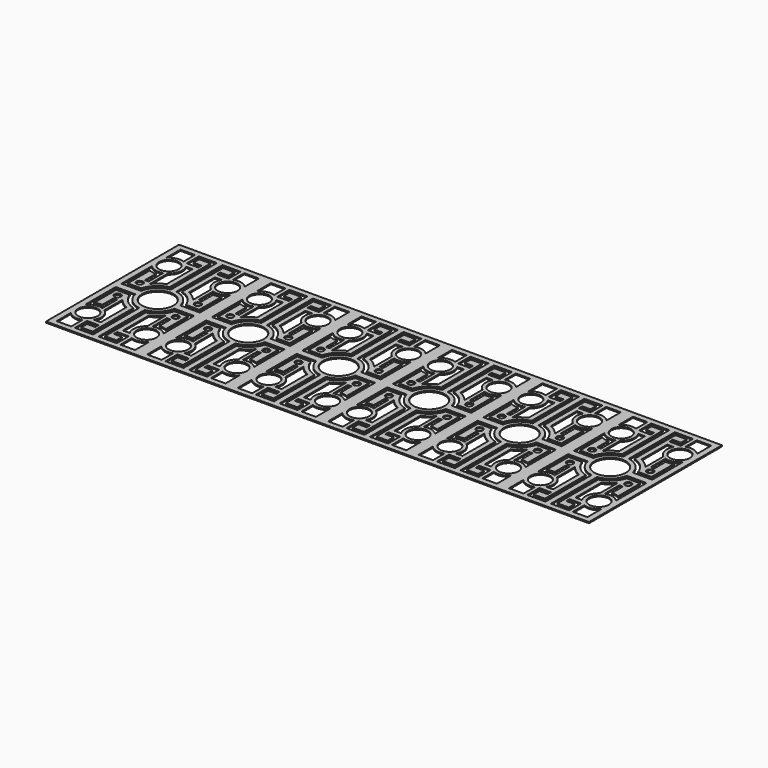
from build123d import *

# Parameters (mm, degrees)
F0_W     = 114.6567612886
F0_H     = 210.6409370899
F0_R     = 12.4910197192
F0_R_2   = 4.1467921194
F1_DEPTH = 1.5


# Not quite as in the source:
# - ends of sketch curves that miss each other by under 0.0002 mm in the source are joined


with BuildPart() as f1:
    # F0 (on Top) → F1 (new body)
    with BuildSketch(Plane.XY):
        with Locations((-114.6567612886, 0)):
            Rectangle(F0_W, F0_H)
        with BuildLine():
            Line((-145.8713209915, -98.179930827), (-164.2948761574, -98.1799308277))
            Line((-164.2948761574, -98.1799308277), (-164.2948761582, -75.6368151295))
            ThreePointArc((-164.2948761582, -75.6368151295), (-155.7558124319, -80.6535810623), (-145.871320992, -80.0372543739))
            Line((-145.871320992, -80.0372543739), (-145.8713209915, -98.179930827))
        make_face(mode=Mode.SUBTRACT)
        with BuildLine():
            Line((-65.0186464199, -98.1799308277), (-83.4422015858, -98.179930827))
            Line((-83.4422015858, -98.179930827), (-83.4422015853, -80.0372543739))
            ThreePointArc((-83.4422015853, -80.0372543739), (-73.5577101454, -80.6535810623), (-65.0187125643, -75.6367543837))
            Line((-65.0187125643, -75.6367543837), (-65.0186464199, -98.1799308277))
        make_face(mode=Mode.SUBTRACT)
        with Locations((-151.8214292036, -64.1815741605)):
            Circle(F0_R, mode=Mode.SUBTRACT)
        with Locations((-77.4920933736, -64.1815741605)):
            Circle(F0_R, mode=Mode.SUBTRACT)
        with BuildLine():
            Line((-118.1285301959, -98.179930827), (-141.0917807374, -98.179930827))
            Line((-141.0917807374, -98.179930827), (-141.0917807374, -79.0647952815))
            Line((-141.0917807374, -79.0647952815), (-126.454948448, -79.0647952815))
            Line((-126.454948448, -79.0647952815), (-126.454948448, -84.2922343872))
            Line((-126.454948448, -84.2922343872), (-136.8864420805, -84.2922343872))
            Line((-136.8864420805, -84.2922343872), (-136.8864420805, -93.5049741529))
            Line((-136.8864420805, -93.5049741529), (-122.577030212, -93.5049741529))
            Line((-122.577030212, -93.5049741529), (-122.4740208728, -28.733128465))
            ThreePointArc((-122.4740208728, -28.733128465), (-135.1857456354, -21.520110379), (-142.9105009887, -9.1127040796))
            Line((-142.9105009887, -9.1127040796), (-160.0093394521, -9.1127040796))
            Line((-160.0093394521, -9.1127040796), (-160.0093394521, -44.1508456133))
            ThreePointArc((-160.0093394521, -44.1508456133), (-155.5141858376, -42.8593906698), (-150.8465334777, -42.5639531376))
            Line((-150.8465334777, -42.5639531376), (-150.8465334777, -25.0186747871))
            Line((-150.8465334777, -25.0186747871), (-146.2718600365, -25.0186747871))
            Line((-146.2718600365, -25.0186747871), (-146.2718600365, -48.3131796792))
            ThreePointArc((-146.2718600365, -48.3131796792), (-155.9772603886, -47.8925370951), (-164.2948761582, -52.9114019158))
            Line((-164.2948761582, -52.9114019158), (-164.2948761582, -4.6059023589))
            Line((-164.2948761582, -4.6059023589), (-139.4034866247, -4.6059023589))
            ThreePointArc((-139.4034866247, -4.6059023589), (-132.0747762414, -18.2690053755), (-118.1285301959, -25.0434131848))
            Line((-118.1285301959, -25.0434131848), (-118.1285301959, -98.179930827))
        make_face(mode=Mode.SUBTRACT)
        with BuildLine():
            Line((-128.7834886465, -72.9014551434), (-137.3203646393, -72.9014551437))
            ThreePointArc((-137.3203646393, -72.9014551437), (-135.2508292753, -60.7563127289), (-141.9659890239, -50.4270295761))
            Line((-141.9659890239, -50.4270295761), (-141.9659890239, -21.7546069546))
            ThreePointArc((-141.9659890239, -21.7546069546), (-135.9951180955, -27.664926491), (-128.7834011022, -31.9747193718))
            Line((-128.7834011022, -31.9747193718), (-128.7834886465, -72.9014551434))
        make_face(mode=Mode.SUBTRACT)
        with BuildLine():
            Line((-92.4270804968, -93.5049741529), (-92.4270804968, -84.2922343872))
            Line((-92.4270804968, -84.2922343872), (-102.8585741293, -84.2922343872))
            Line((-102.8585741293, -84.2922343872), (-102.8585741293, -79.0647952815))
            Line((-102.8585741293, -79.0647952815), (-88.2217418399, -79.0647952815))
            Line((-88.2217418399, -79.0647952815), (-88.2217418399, -98.179930827))
            Line((-88.2217418399, -98.179930827), (-111.1849923813, -98.179930827))
            Line((-111.1849923813, -98.179930827), (-111.1849923813, -25.0434131848))
            ThreePointArc((-111.1849923813, -25.0434131848), (-97.2387463359, -18.2690053755), (-89.9100359526, -4.6059023589))
            Line((-89.9100359526, -4.6059023589), (-65.018646419, -4.6059023589))
            Line((-65.018646419, -4.6059023589), (-65.018646419, -52.9114019158))
            ThreePointArc((-65.018646419, -52.9114019158), (-73.3362621887, -47.8925370951), (-83.0416625408, -48.3131796792))
            Line((-83.0416625408, -48.3131796792), (-83.0416625408, -25.0186747871))
            Line((-83.0416625408, -25.0186747871), (-78.4669890996, -25.0186747871))
            Line((-78.4669890996, -25.0186747871), (-78.4669890996, -42.5639531376))
            ThreePointArc((-78.4669890996, -42.5639531376), (-73.7993367396, -42.8593906698), (-69.3041831251, -44.1508456133))
            Line((-69.3041831251, -44.1508456133), (-69.3041831251, -9.1127040796))
            Line((-69.3041831251, -9.1127040796), (-86.4030215886, -9.1127040796))
            ThreePointArc((-86.4030215886, -9.1127040796), (-94.1277769419, -21.520110379), (-106.8395017045, -28.733128465))
            Line((-106.8395017045, -28.733128465), (-106.7364923652, -93.5049741529))
            Line((-106.7364923652, -93.5049741529), (-92.4270804968, -93.5049741529))
        make_face(mode=Mode.SUBTRACT)
        with BuildLine():
            ThreePointArc((-87.3475335534, -50.4270295761), (-94.062693302, -60.7563127289), (-91.993157938, -72.9014551437))
            Line((-91.993157938, -72.9014551437), (-100.5300339308, -72.9014551434))
            Line((-100.5300339308, -72.9014551434), (-100.5300339308, -31.9747193718))
            ThreePointArc((-100.5300339308, -31.9747193718), (-93.3184044818, -27.664926491), (-87.3475335534, -21.7546069546))
            Line((-87.3475335534, -21.7546069546), (-87.3475335534, -50.4270295761))
        make_face(mode=Mode.SUBTRACT)
        with Locations((-151.4818519357, -17.5733412616)):
            Circle(F0_R_2, mode=Mode.SUBTRACT)
        with Locations((-77.8316706415, -17.5733412616)):
            Circle(F0_R_2, mode=Mode.SUBTRACT)
        with BuildLine():
            ThreePointArc((-134.3588686144, 2.5716374978), (-114.6567612886, 19.8692313011), (-94.9546539628, 2.5716374978))
            ThreePointArc((-94.9546539628, 2.5716374978), (-94.8172855837, 1.2286792521), (-94.7714255579, -0.1205070876))
            ThreePointArc((-94.7714255579, -0.1205070876), (-100.5966835989, -14.1758679), (-114.6567612886, -19.9897318622))
            ThreePointArc((-114.6567612886, -19.9897318622), (-129.6388295453, -13.1897947203), (-134.3588686144, 2.5716374978))
        make_face(mode=Mode.SUBTRACT)
        with Locations((-151.4979563653, 17.452834174)):
            Circle(F0_R_2, mode=Mode.SUBTRACT)
        with Locations((-77.8155662119, 17.452834174)):
            Circle(F0_R_2, mode=Mode.SUBTRACT)
        with BuildLine():
            ThreePointArc((-141.9820934535, 50.3065224885), (-135.2669337049, 60.6358056413), (-137.3364690689, 72.7809480561))
            Line((-137.3364690689, 72.7809480561), (-128.7995930761, 72.7809480559))
            Line((-128.7995930761, 72.7809480559), (-128.7995930761, 31.8542122842))
            ThreePointArc((-128.7995930761, 31.8542122842), (-136.0112225251, 27.5444194035), (-141.9820934535, 21.634099867))
            Line((-141.9820934535, 21.634099867), (-141.9820934535, 50.3065224885))
        make_face(mode=Mode.SUBTRACT)
        with BuildLine():
            Line((-136.9025465101, 93.3844670653), (-136.9025465101, 84.1717272997))
            Line((-136.9025465101, 84.1717272997), (-126.4710528776, 84.1717272997))
            Line((-126.4710528776, 84.1717272997), (-126.4710528776, 78.9442881942))
            Line((-126.4710528776, 78.9442881942), (-141.107885167, 78.9442881942))
            Line((-141.107885167, 78.9442881942), (-141.107885167, 98.0594237397))
            Line((-141.107885167, 98.0594237397), (-118.1446346255, 98.0594237397))
            Line((-118.1446346255, 98.0594237397), (-118.1446346255, 24.9229060972))
            ThreePointArc((-118.1446346255, 24.9229060972), (-132.090880671, 18.1484982879), (-139.4195910543, 4.4853952713))
            Line((-139.4195910543, 4.4853952713), (-164.3109805878, 4.4853952713))
            Line((-164.3109805878, 4.4853952713), (-164.3109805878, 52.7908948282))
            ThreePointArc((-164.3109805878, 52.7908948282), (-155.9933648182, 47.7720300076), (-146.2879644661, 48.1926725917))
            Line((-146.2879644661, 48.1926725917), (-146.2879644661, 24.8981676996))
            Line((-146.2879644661, 24.8981676996), (-150.8626379073, 24.8981676996))
            Line((-150.8626379073, 24.8981676996), (-150.8626379073, 42.44344605))
            ThreePointArc((-150.8626379073, 42.44344605), (-155.5302902672, 42.7388835823), (-160.0254438818, 44.0303385258))
            Line((-160.0254438818, 44.0303385258), (-160.0254438818, 8.992196992))
            Line((-160.0254438818, 8.992196992), (-142.9266054183, 8.992196992))
            ThreePointArc((-142.9266054183, 8.992196992), (-135.201850065, 21.3996032915), (-122.4901253024, 28.6126213774))
            Line((-122.4901253024, 28.6126213774), (-122.5931346416, 93.3844670653))
            Line((-122.5931346416, 93.3844670653), (-136.9025465101, 93.3844670653))
        make_face(mode=Mode.SUBTRACT)
        with BuildLine():
            Line((-100.5139295012, 72.7809480559), (-91.9770535084, 72.7809480561))
            ThreePointArc((-91.9770535084, 72.7809480561), (-94.0465888724, 60.6358056413), (-87.3314291238, 50.3065224885))
            Line((-87.3314291238, 50.3065224885), (-87.3314291238, 21.634099867))
            ThreePointArc((-87.3314291238, 21.634099867), (-93.3023000522, 27.5444194035), (-100.5140170454, 31.8542122842))
            Line((-100.5140170454, 31.8542122842), (-100.5139295012, 72.7809480559))
        make_face(mode=Mode.SUBTRACT)
        with BuildLine():
            Line((-111.1688879517, 98.0594237397), (-88.2056374103, 98.0594237397))
            Line((-88.2056374103, 98.0594237397), (-88.2056374103, 78.9442881942))
            Line((-88.2056374103, 78.9442881942), (-102.8424696997, 78.9442881942))
            Line((-102.8424696997, 78.9442881942), (-102.8424696997, 84.1717272997))
            Line((-102.8424696997, 84.1717272997), (-92.4109760672, 84.1717272997))
            Line((-92.4109760672, 84.1717272997), (-92.4109760672, 93.3844670653))
            Line((-92.4109760672, 93.3844670653), (-106.7203879356, 93.3844670653))
            Line((-106.7203879356, 93.3844670653), (-106.8233972749, 28.6126213774))
            ThreePointArc((-106.8233972749, 28.6126213774), (-94.1116725123, 21.3996032915), (-86.386917159, 8.992196992))
            Line((-86.386917159, 8.992196992), (-69.2880786955, 8.992196992))
            Line((-69.2880786955, 8.992196992), (-69.2880786955, 44.0303385258))
            ThreePointArc((-69.2880786955, 44.0303385258), (-73.78323231, 42.7388835823), (-78.45088467, 42.44344605))
            Line((-78.45088467, 42.44344605), (-78.45088467, 24.8981676996))
            Line((-78.45088467, 24.8981676996), (-83.0255581112, 24.8981676996))
            Line((-83.0255581112, 24.8981676996), (-83.0255581112, 48.1926725917))
            ThreePointArc((-83.0255581112, 48.1926725917), (-73.3201577591, 47.7720300076), (-65.0025419894, 52.7908948282))
            Line((-65.0025419894, 52.7908948282), (-65.0025419894, 4.4853952713))
            Line((-65.0025419894, 4.4853952713), (-89.893931523, 4.4853952713))
            ThreePointArc((-89.893931523, 4.4853952713), (-97.2226419063, 18.1484982879), (-111.1688879517, 24.9229060972))
            Line((-111.1688879517, 24.9229060972), (-111.1688879517, 98.0594237397))
        make_face(mode=Mode.SUBTRACT)
        with Locations((-151.8375336332, 64.0610670729)):
            Circle(F0_R, mode=Mode.SUBTRACT)
        with Locations((-77.475988944, 64.0610670729)):
            Circle(F0_R, mode=Mode.SUBTRACT)
        with BuildLine():
            Line((-164.3109805878, 75.516308042), (-164.3109805873, 98.0594237402))
            Line((-164.3109805873, 98.0594237402), (-145.8874254222, 98.0594237397))
            Line((-145.8874254222, 98.0594237397), (-145.8874254226, 79.9167472867))
            ThreePointArc((-145.8874254226, 79.9167472867), (-155.771916862, 80.5330739746), (-164.3109805878, 75.516308042))
        make_face(mode=Mode.SUBTRACT)
        with BuildLine():
            Line((-83.4260971551, 98.0594237397), (-65.00254199, 98.0594237402))
            Line((-65.00254199, 98.0594237402), (-65.0025419894, 75.516308042))
            ThreePointArc((-65.0025419894, 75.516308042), (-73.5416057152, 80.5330739746), (-83.4260971547, 79.9167472867))
            Line((-83.4260971547, 79.9167472867), (-83.4260971551, 98.0594237397))
        make_face(mode=Mode.SUBTRACT)
        with Locations((229.3135225773, 0)):
            Rectangle(F0_W, F0_H)
        with BuildLine():
            Line((198.0989628739, -80.0372543739), (198.0989628744, -98.179930827))
            Line((198.0989628744, -98.179930827), (179.6754077085, -98.1799308277))
            Line((179.6754077085, -98.1799308277), (179.6754077077, -75.6368151295))
            ThreePointArc((179.6754077077, -75.6368151295), (188.214471434, -80.6535810623), (198.0989628739, -80.0372543739))
        make_face(mode=Mode.SUBTRACT)
        with BuildLine():
            Line((278.9516374469, -75.6368151295), (278.951637446, -98.1799308277))
            Line((278.951637446, -98.1799308277), (260.5280822802, -98.179930827))
            Line((260.5280822802, -98.179930827), (260.5280822806, -80.0372543739))
            ThreePointArc((260.5280822806, -80.0372543739), (270.4125737205, -80.6535810623), (278.9516374469, -75.6368151295))
        make_face(mode=Mode.SUBTRACT)
        with Locations((192.1488546623, -64.1815741605)):
            Circle(F0_R, mode=Mode.SUBTRACT)
        with Locations((266.4781904923, -64.1815741605)):
            Circle(F0_R, mode=Mode.SUBTRACT)
        with BuildLine():
            ThreePointArc((197.6984238295, -48.3131796792), (187.9930234773, -47.8925370951), (179.6754077077, -52.9114019158))
            Line((179.6754077077, -52.9114019158), (179.6754077077, -4.6059023589))
            Line((179.6754077077, -4.6059023589), (204.5667972412, -4.6059023589))
            ThreePointArc((204.5667972412, -4.6059023589), (211.8955076246, -18.2690053755), (225.84175367, -25.0434131848))
            Line((225.84175367, -25.0434131848), (225.84175367, -98.179930827))
            Line((225.84175367, -98.179930827), (202.8785031285, -98.179930827))
            Line((202.8785031285, -98.179930827), (202.8785031285, -79.0647952815))
            Line((202.8785031285, -79.0647952815), (217.5153354179, -79.0647952815))
            Line((217.5153354179, -79.0647952815), (217.5153354179, -84.2922343872))
            Line((217.5153354179, -84.2922343872), (207.0838417854, -84.2922343872))
            Line((207.0838417854, -84.2922343872), (207.0838417854, -93.5049741529))
            Line((207.0838417854, -93.5049741529), (221.3932536539, -93.5049741529))
            Line((221.3932536539, -93.5049741529), (221.4962629932, -28.733128465))
            ThreePointArc((221.4962629932, -28.733128465), (208.7845382306, -21.520110379), (201.0597828772, -9.1127040796))
            Line((201.0597828772, -9.1127040796), (183.9609444138, -9.1127040796))
            Line((183.9609444138, -9.1127040796), (183.9609444138, -44.1508456133))
            ThreePointArc((183.9609444138, -44.1508456133), (188.4560980283, -42.8593906698), (193.1237503883, -42.5639531376))
            Line((193.1237503883, -42.5639531376), (193.1237503883, -25.0186747871))
            Line((193.1237503883, -25.0186747871), (197.6984238295, -25.0186747871))
            Line((197.6984238295, -25.0186747871), (197.6984238295, -48.3131796792))
        make_face(mode=Mode.SUBTRACT)
        with BuildLine():
            Line((215.1867952194, -72.9014551434), (206.6499192266, -72.9014551437))
            ThreePointArc((206.6499192266, -72.9014551437), (208.7194545906, -60.7563127289), (202.004294842, -50.4270295761))
            Line((202.004294842, -50.4270295761), (202.004294842, -21.7546069546))
            ThreePointArc((202.004294842, -21.7546069546), (207.9751657704, -27.664926491), (215.1868827637, -31.9747193718))
            Line((215.1868827637, -31.9747193718), (215.1867952194, -72.9014551434))
        make_face(mode=Mode.SUBTRACT)
        with BuildLine():
            Line((260.9286213251, -48.3131796792), (260.9286213251, -25.0186747871))
            Line((260.9286213251, -25.0186747871), (265.5032947663, -25.0186747871))
            Line((265.5032947663, -25.0186747871), (265.5032947663, -42.5639531376))
            ThreePointArc((265.5032947663, -42.5639531376), (270.1709471263, -42.8593906698), (274.6661007408, -44.1508456133))
            Line((274.6661007408, -44.1508456133), (274.6661007408, -9.1127040796))
            Line((274.6661007408, -9.1127040796), (257.5672622774, -9.1127040796))
            ThreePointArc((257.5672622774, -9.1127040796), (249.842506924, -21.520110379), (237.1307821614, -28.733128465))
            Line((237.1307821614, -28.733128465), (237.2337915007, -93.5049741529))
            Line((237.2337915007, -93.5049741529), (251.5432033691, -93.5049741529))
            Line((251.5432033691, -93.5049741529), (251.5432033691, -84.2922343872))
            Line((251.5432033691, -84.2922343872), (241.1117097366, -84.2922343872))
            Line((241.1117097366, -84.2922343872), (241.1117097366, -79.0647952815))
            Line((241.1117097366, -79.0647952815), (255.748542026, -79.0647952815))
            Line((255.748542026, -79.0647952815), (255.748542026, -98.179930827))
            Line((255.748542026, -98.179930827), (232.7852914846, -98.179930827))
            Line((232.7852914846, -98.179930827), (232.7852914846, -25.0434131848))
            ThreePointArc((232.7852914846, -25.0434131848), (246.73153753, -18.2690053755), (254.0602479134, -4.6059023589))
            Line((254.0602479134, -4.6059023589), (278.9516374469, -4.6059023589))
            Line((278.9516374469, -4.6059023589), (278.9516374469, -52.9114019158))
            ThreePointArc((278.9516374469, -52.9114019158), (270.6340216773, -47.8925370951), (260.9286213251, -48.3131796792))
        make_face(mode=Mode.SUBTRACT)
        with BuildLine():
            ThreePointArc((256.6227503125, -50.4270295761), (249.9075905639, -60.7563127289), (251.9771259279, -72.9014551437))
            Line((251.9771259279, -72.9014551437), (243.4402499351, -72.9014551434))
            Line((243.4402499351, -72.9014551434), (243.4402499351, -31.9747193718))
            ThreePointArc((243.4402499351, -31.9747193718), (250.6518793842, -27.664926491), (256.6227503125, -21.7546069546))
            Line((256.6227503125, -21.7546069546), (256.6227503125, -50.4270295761))
        make_face(mode=Mode.SUBTRACT)
        with Locations((192.4884319302, -17.5733412616)):
            Circle(F0_R_2, mode=Mode.SUBTRACT)
        with Locations((266.1386132244, -17.5733412616)):
            Circle(F0_R_2, mode=Mode.SUBTRACT)
        with BuildLine():
            ThreePointArc((249.0156299031, 2.5716374978), (249.1529982822, 1.2286792521), (249.198858308, -0.1205070876))
            ThreePointArc((249.198858308, -0.1205070876), (243.373600267, -14.1758679), (229.3135225773, -19.9897318622))
            ThreePointArc((229.3135225773, -19.9897318622), (214.3314543207, -13.1897947203), (209.6114152515, 2.5716374978))
            ThreePointArc((209.6114152515, 2.5716374978), (229.3135225773, 19.8692313011), (249.0156299031, 2.5716374978))
        make_face(mode=Mode.SUBTRACT)
        with Locations((192.4723275006, 17.452834174)):
            Circle(F0_R_2, mode=Mode.SUBTRACT)
        with Locations((266.154717654, 17.452834174)):
            Circle(F0_R_2, mode=Mode.SUBTRACT)
        with BuildLine():
            ThreePointArc((201.9881904124, 50.3065224885), (208.703350161, 60.6358056413), (206.633814797, 72.7809480561))
            Line((206.633814797, 72.7809480561), (215.1706907898, 72.7809480559))
            Line((215.1706907898, 72.7809480559), (215.1706907898, 31.8542122842))
            ThreePointArc((215.1706907898, 31.8542122842), (207.9590613408, 27.5444194035), (201.9881904124, 21.634099867))
            Line((201.9881904124, 21.634099867), (201.9881904124, 50.3065224885))
        make_face(mode=Mode.SUBTRACT)
        with BuildLine():
            Line((197.6823193999, 48.1926725917), (197.6823193999, 24.8981676996))
            Line((197.6823193999, 24.8981676996), (193.1076459587, 24.8981676996))
            Line((193.1076459587, 24.8981676996), (193.1076459587, 42.44344605))
            ThreePointArc((193.1076459587, 42.44344605), (188.4399935987, 42.7388835823), (183.9448399842, 44.0303385258))
            Line((183.9448399842, 44.0303385258), (183.9448399842, 8.992196992))
            Line((183.9448399842, 8.992196992), (201.0436784476, 8.992196992))
            ThreePointArc((201.0436784476, 8.992196992), (208.768433801, 21.3996032915), (221.4801585636, 28.6126213774))
            Line((221.4801585636, 28.6126213774), (221.3771492243, 93.3844670653))
            Line((221.3771492243, 93.3844670653), (207.0677373558, 93.3844670653))
            Line((207.0677373558, 93.3844670653), (207.0677373558, 84.1717272997))
            Line((207.0677373558, 84.1717272997), (217.4992309883, 84.1717272997))
            Line((217.4992309883, 84.1717272997), (217.4992309883, 78.9442881942))
            Line((217.4992309883, 78.9442881942), (202.8623986989, 78.9442881942))
            Line((202.8623986989, 78.9442881942), (202.8623986989, 98.0594237397))
            Line((202.8623986989, 98.0594237397), (225.8256492404, 98.0594237397))
            Line((225.8256492404, 98.0594237397), (225.8256492404, 24.9229060972))
            ThreePointArc((225.8256492404, 24.9229060972), (211.879403195, 18.1484982879), (204.5506928116, 4.4853952713))
            Line((204.5506928116, 4.4853952713), (179.6593032781, 4.4853952713))
            Line((179.6593032781, 4.4853952713), (179.6593032781, 52.7908948282))
            ThreePointArc((179.6593032781, 52.7908948282), (187.9769190477, 47.7720300076), (197.6823193999, 48.1926725917))
        make_face(mode=Mode.SUBTRACT)
        with BuildLine():
            Line((243.4563543647, 72.7809480559), (251.9932303575, 72.7809480561))
            ThreePointArc((251.9932303575, 72.7809480561), (249.9236949935, 60.6358056413), (256.6388547421, 50.3065224885))
            Line((256.6388547421, 50.3065224885), (256.6388547421, 21.634099867))
            ThreePointArc((256.6388547421, 21.634099867), (250.6679838138, 27.5444194035), (243.4562668205, 31.8542122842))
            Line((243.4562668205, 31.8542122842), (243.4563543647, 72.7809480559))
        make_face(mode=Mode.SUBTRACT)
        with BuildLine():
            ThreePointArc((274.6822051704, 44.0303385258), (270.1870515559, 42.7388835823), (265.5193991959, 42.44344605))
            Line((265.5193991959, 42.44344605), (265.5193991959, 24.8981676996))
            Line((265.5193991959, 24.8981676996), (260.9447257547, 24.8981676996))
            Line((260.9447257547, 24.8981676996), (260.9447257547, 48.1926725917))
            ThreePointArc((260.9447257547, 48.1926725917), (270.6501261069, 47.7720300076), (278.9677418765, 52.7908948282))
            Line((278.9677418765, 52.7908948282), (278.9677418765, 4.4853952713))
            Line((278.9677418765, 4.4853952713), (254.076352343, 4.4853952713))
            ThreePointArc((254.076352343, 4.4853952713), (246.7476419596, 18.1484982879), (232.8013959142, 24.9229060972))
            Line((232.8013959142, 24.9229060972), (232.8013959142, 98.0594237397))
            Line((232.8013959142, 98.0594237397), (255.7646464556, 98.0594237397))
            Line((255.7646464556, 98.0594237397), (255.7646464556, 78.9442881942))
            Line((255.7646464556, 78.9442881942), (241.1278141662, 78.9442881942))
            Line((241.1278141662, 78.9442881942), (241.1278141662, 84.1717272997))
            Line((241.1278141662, 84.1717272997), (251.5593077987, 84.1717272997))
            Line((251.5593077987, 84.1717272997), (251.5593077987, 93.3844670653))
            Line((251.5593077987, 93.3844670653), (237.2498959303, 93.3844670653))
            Line((237.2498959303, 93.3844670653), (237.146886591, 28.6126213774))
            ThreePointArc((237.146886591, 28.6126213774), (249.8586113536, 21.3996032915), (257.583366707, 8.992196992))
            Line((257.583366707, 8.992196992), (274.6822051704, 8.992196992))
            Line((274.6822051704, 8.992196992), (274.6822051704, 44.0303385258))
        make_face(mode=Mode.SUBTRACT)
        with Locations((192.1327502327, 64.0610670729)):
            Circle(F0_R, mode=Mode.SUBTRACT)
        with Locations((266.4942949219, 64.0610670729)):
            Circle(F0_R, mode=Mode.SUBTRACT)
        with BuildLine():
            ThreePointArc((198.0828584433, 79.9167472867), (188.1983670039, 80.5330739746), (179.6593694234, 75.5162472961))
            Line((179.6593694234, 75.5162472961), (179.6593032786, 98.0594237402))
            Line((179.6593032786, 98.0594237402), (198.0828584438, 98.0594237397))
            Line((198.0828584438, 98.0594237397), (198.0828584433, 79.9167472867))
        make_face(mode=Mode.SUBTRACT)
        with BuildLine():
            Line((260.5441867108, 98.0594237397), (278.9677418759, 98.0594237402))
            Line((278.9677418759, 98.0594237402), (278.9677418765, 75.516308042))
            ThreePointArc((278.9677418765, 75.516308042), (270.4286781507, 80.5330739746), (260.5441867113, 79.9167472867))
            Line((260.5441867113, 79.9167472867), (260.5441867108, 98.0594237397))
        make_face(mode=Mode.SUBTRACT)
        with Locations((114.6567612886, 0)):
            Rectangle(F0_W, F0_H)
        with BuildLine():
            Line((83.4422015858, -98.179930827), (65.0186464199, -98.1799308277))
            Line((65.0186464199, -98.1799308277), (65.018646419, -75.6368151295))
            ThreePointArc((65.018646419, -75.6368151295), (73.5577101454, -80.6535810623), (83.4422015853, -80.0372543739))
            Line((83.4422015853, -80.0372543739), (83.4422015858, -98.179930827))
        make_face(mode=Mode.SUBTRACT)
        with Locations((77.4920933736, -64.1815741605)):
            Circle(F0_R, mode=Mode.SUBTRACT)
        with BuildLine():
            Line((164.2948761574, -98.1799308277), (145.8713209915, -98.179930827))
            Line((145.8713209915, -98.179930827), (145.871320992, -80.0372543739))
            ThreePointArc((145.871320992, -80.0372543739), (155.7558124319, -80.6535810623), (164.294810013, -75.6367543837))
            Line((164.294810013, -75.6367543837), (164.2948761574, -98.1799308277))
        make_face(mode=Mode.SUBTRACT)
        with Locations((151.8214292036, -64.1815741605)):
            Circle(F0_R, mode=Mode.SUBTRACT)
        with BuildLine():
            Line((102.8585741293, -84.2922343872), (92.4270804968, -84.2922343872))
            Line((92.4270804968, -84.2922343872), (92.4270804968, -93.5049741529))
            Line((92.4270804968, -93.5049741529), (106.7364923652, -93.5049741529))
            Line((106.7364923652, -93.5049741529), (106.8395017045, -28.733128465))
            ThreePointArc((106.8395017045, -28.733128465), (94.1277769419, -21.520110379), (86.4030215886, -9.1127040796))
            Line((86.4030215886, -9.1127040796), (69.3041831251, -9.1127040796))
            Line((69.3041831251, -9.1127040796), (69.3041831251, -44.1508456133))
            ThreePointArc((69.3041831251, -44.1508456133), (73.7993367396, -42.8593906698), (78.4669890996, -42.5639531376))
            Line((78.4669890996, -42.5639531376), (78.4669890996, -25.0186747871))
            Line((78.4669890996, -25.0186747871), (83.0416625408, -25.0186747871))
            Line((83.0416625408, -25.0186747871), (83.0416625408, -48.3131796792))
            ThreePointArc((83.0416625408, -48.3131796792), (73.3362621887, -47.8925370951), (65.018646419, -52.9114019158))
            Line((65.018646419, -52.9114019158), (65.018646419, -4.6059023589))
            Line((65.018646419, -4.6059023589), (89.9100359526, -4.6059023589))
            ThreePointArc((89.9100359526, -4.6059023589), (97.2387463359, -18.2690053755), (111.1849923813, -25.0434131848))
            Line((111.1849923813, -25.0434131848), (111.1849923813, -98.179930827))
            Line((111.1849923813, -98.179930827), (88.2217418399, -98.179930827))
            Line((88.2217418399, -98.179930827), (88.2217418399, -79.0647952815))
            Line((88.2217418399, -79.0647952815), (102.8585741293, -79.0647952815))
            Line((102.8585741293, -79.0647952815), (102.8585741293, -84.2922343872))
        make_face(mode=Mode.SUBTRACT)
        with BuildLine():
            Line((100.5300339308, -72.9014551434), (91.993157938, -72.9014551437))
            ThreePointArc((91.993157938, -72.9014551437), (94.062693302, -60.7563127289), (87.3475335534, -50.4270295761))
            Line((87.3475335534, -50.4270295761), (87.3475335534, -21.7546069546))
            ThreePointArc((87.3475335534, -21.7546069546), (93.3184044818, -27.664926491), (100.5301214751, -31.9747193718))
            Line((100.5301214751, -31.9747193718), (100.5300339308, -72.9014551434))
        make_face(mode=Mode.SUBTRACT)
        with Locations((77.8316706415, -17.5733412616)):
            Circle(F0_R_2, mode=Mode.SUBTRACT)
        with BuildLine():
            ThreePointArc((141.9659890239, -50.4270295761), (135.2508292753, -60.7563127289), (137.3203646393, -72.9014551437))
            Line((137.3203646393, -72.9014551437), (128.7834886465, -72.9014551434))
            Line((128.7834886465, -72.9014551434), (128.7834886465, -31.9747193718))
            ThreePointArc((128.7834886465, -31.9747193718), (135.9951180955, -27.664926491), (141.9659890239, -21.7546069546))
            Line((141.9659890239, -21.7546069546), (141.9659890239, -50.4270295761))
        make_face(mode=Mode.SUBTRACT)
        with BuildLine():
            Line((136.8864420805, -84.2922343872), (126.454948448, -84.2922343872))
            Line((126.454948448, -84.2922343872), (126.454948448, -79.0647952815))
            Line((126.454948448, -79.0647952815), (141.0917807374, -79.0647952815))
            Line((141.0917807374, -79.0647952815), (141.0917807374, -98.179930827))
            Line((141.0917807374, -98.179930827), (118.1285301959, -98.179930827))
            Line((118.1285301959, -98.179930827), (118.1285301959, -25.0434131848))
            ThreePointArc((118.1285301959, -25.0434131848), (132.0747762414, -18.2690053755), (139.4034866247, -4.6059023589))
            Line((139.4034866247, -4.6059023589), (164.2948761582, -4.6059023589))
            Line((164.2948761582, -4.6059023589), (164.2948761582, -52.9114019158))
            ThreePointArc((164.2948761582, -52.9114019158), (155.9772603886, -47.8925370951), (146.2718600365, -48.3131796792))
            Line((146.2718600365, -48.3131796792), (146.2718600365, -25.0186747871))
            Line((146.2718600365, -25.0186747871), (150.8465334777, -25.0186747871))
            Line((150.8465334777, -25.0186747871), (150.8465334777, -42.5639531376))
            ThreePointArc((150.8465334777, -42.5639531376), (155.5141858376, -42.8593906698), (160.0093394521, -44.1508456133))
            Line((160.0093394521, -44.1508456133), (160.0093394521, -9.1127040796))
            Line((160.0093394521, -9.1127040796), (142.9105009887, -9.1127040796))
            ThreePointArc((142.9105009887, -9.1127040796), (135.1857456354, -21.520110379), (122.4740208728, -28.733128465))
            Line((122.4740208728, -28.733128465), (122.577030212, -93.5049741529))
            Line((122.577030212, -93.5049741529), (136.8864420805, -93.5049741529))
            Line((136.8864420805, -93.5049741529), (136.8864420805, -84.2922343872))
        make_face(mode=Mode.SUBTRACT)
        with Locations((151.4818519357, -17.5733412616)):
            Circle(F0_R_2, mode=Mode.SUBTRACT)
        with BuildLine():
            ThreePointArc((94.9546539628, 2.5716374978), (114.6567612886, 19.8692313011), (134.3588686144, 2.5716374978))
            ThreePointArc((134.3588686144, 2.5716374978), (134.4962369936, 1.2286792521), (134.5420970194, -0.1205070876))
            ThreePointArc((134.5420970194, -0.1205070876), (128.7168389784, -14.1758679), (114.6567612886, -19.9897318622))
            ThreePointArc((114.6567612886, -19.9897318622), (99.674693032, -13.1897947203), (94.9546539628, 2.5716374978))
        make_face(mode=Mode.SUBTRACT)
        with Locations((77.8155662119, 17.452834174)):
            Circle(F0_R_2, mode=Mode.SUBTRACT)
        with BuildLine():
            Line((102.8424696997, 84.1717272997), (102.8424696997, 78.9442881942))
            Line((102.8424696997, 78.9442881942), (88.2056374103, 78.9442881942))
            Line((88.2056374103, 78.9442881942), (88.2056374103, 98.0594237397))
            Line((88.2056374103, 98.0594237397), (111.1688879517, 98.0594237397))
            Line((111.1688879517, 98.0594237397), (111.1688879517, 24.9229060972))
            ThreePointArc((111.1688879517, 24.9229060972), (97.2226419063, 18.1484982879), (89.893931523, 4.4853952713))
            Line((89.893931523, 4.4853952713), (65.0025419894, 4.4853952713))
            Line((65.0025419894, 4.4853952713), (65.0025419894, 52.7908948282))
            ThreePointArc((65.0025419894, 52.7908948282), (73.3201577591, 47.7720300076), (83.0255581112, 48.1926725917))
            Line((83.0255581112, 48.1926725917), (83.0255581112, 24.8981676996))
            Line((83.0255581112, 24.8981676996), (78.45088467, 24.8981676996))
            Line((78.45088467, 24.8981676996), (78.45088467, 42.44344605))
            ThreePointArc((78.45088467, 42.44344605), (73.78323231, 42.7388835823), (69.2880786955, 44.0303385258))
            Line((69.2880786955, 44.0303385258), (69.2880786955, 8.992196992))
            Line((69.2880786955, 8.992196992), (86.386917159, 8.992196992))
            ThreePointArc((86.386917159, 8.992196992), (94.1116725123, 21.3996032915), (106.8233972749, 28.6126213774))
            Line((106.8233972749, 28.6126213774), (106.7203879356, 93.3844670653))
            Line((106.7203879356, 93.3844670653), (92.4109760672, 93.3844670653))
            Line((92.4109760672, 93.3844670653), (92.4109760672, 84.1717272997))
            Line((92.4109760672, 84.1717272997), (102.8424696997, 84.1717272997))
        make_face(mode=Mode.SUBTRACT)
        with BuildLine():
            ThreePointArc((87.3314291238, 50.3065224885), (94.0465888724, 60.6358056413), (91.9770535084, 72.7809480561))
            Line((91.9770535084, 72.7809480561), (100.5139295012, 72.7809480559))
            Line((100.5139295012, 72.7809480559), (100.5139295012, 31.8542122842))
            ThreePointArc((100.5139295012, 31.8542122842), (93.3023000522, 27.5444194035), (87.3314291238, 21.634099867))
            Line((87.3314291238, 21.634099867), (87.3314291238, 50.3065224885))
        make_face(mode=Mode.SUBTRACT)
        with Locations((151.4979563653, 17.452834174)):
            Circle(F0_R_2, mode=Mode.SUBTRACT)
        with BuildLine():
            Line((128.7995930761, 72.7809480559), (137.3364690689, 72.7809480561))
            ThreePointArc((137.3364690689, 72.7809480561), (135.2669337049, 60.6358056413), (141.9820934535, 50.3065224885))
            Line((141.9820934535, 50.3065224885), (141.9820934535, 21.634099867))
            ThreePointArc((141.9820934535, 21.634099867), (136.0112225251, 27.5444194035), (128.7995055318, 31.8542122842))
            Line((128.7995055318, 31.8542122842), (128.7995930761, 72.7809480559))
        make_face(mode=Mode.SUBTRACT)
        with BuildLine():
            Line((126.4710528776, 78.9442881942), (126.4710528776, 84.1717272997))
            Line((126.4710528776, 84.1717272997), (136.9025465101, 84.1717272997))
            Line((136.9025465101, 84.1717272997), (136.9025465101, 93.3844670653))
            Line((136.9025465101, 93.3844670653), (122.5931346416, 93.3844670653))
            Line((122.5931346416, 93.3844670653), (122.4901253024, 28.6126213774))
            ThreePointArc((122.4901253024, 28.6126213774), (135.201850065, 21.3996032915), (142.9266054183, 8.992196992))
            Line((142.9266054183, 8.992196992), (160.0254438818, 8.992196992))
            Line((160.0254438818, 8.992196992), (160.0254438818, 44.0303385258))
            ThreePointArc((160.0254438818, 44.0303385258), (155.5302902672, 42.7388835823), (150.8626379073, 42.44344605))
            Line((150.8626379073, 42.44344605), (150.8626379073, 24.8981676996))
            Line((150.8626379073, 24.8981676996), (146.2879644661, 24.8981676996))
            Line((146.2879644661, 24.8981676996), (146.2879644661, 48.1926725917))
            ThreePointArc((146.2879644661, 48.1926725917), (155.9933648182, 47.7720300076), (164.3109805878, 52.7908948282))
            Line((164.3109805878, 52.7908948282), (164.3109805878, 4.4853952713))
            Line((164.3109805878, 4.4853952713), (139.4195910543, 4.4853952713))
            ThreePointArc((139.4195910543, 4.4853952713), (132.090880671, 18.1484982879), (118.1446346255, 24.9229060972))
            Line((118.1446346255, 24.9229060972), (118.1446346255, 98.0594237397))
            Line((118.1446346255, 98.0594237397), (141.107885167, 98.0594237397))
            Line((141.107885167, 98.0594237397), (141.107885167, 78.9442881942))
            Line((141.107885167, 78.9442881942), (126.4710528776, 78.9442881942))
        make_face(mode=Mode.SUBTRACT)
        with Locations((77.475988944, 64.0610670729)):
            Circle(F0_R, mode=Mode.SUBTRACT)
        with BuildLine():
            Line((65.0025419894, 75.516308042), (65.00254199, 98.0594237402))
            Line((65.00254199, 98.0594237402), (83.4260971551, 98.0594237397))
            Line((83.4260971551, 98.0594237397), (83.4260971547, 79.9167472867))
            ThreePointArc((83.4260971547, 79.9167472867), (73.5416057152, 80.5330739746), (65.0025419894, 75.516308042))
        make_face(mode=Mode.SUBTRACT)
        with Locations((151.8375336332, 64.0610670729)):
            Circle(F0_R, mode=Mode.SUBTRACT)
        with BuildLine():
            Line((164.3109805873, 98.0594237402), (164.3109805878, 75.516308042))
            ThreePointArc((164.3109805878, 75.516308042), (155.771916862, 80.5330739746), (145.8874254226, 79.9167472867))
            Line((145.8874254226, 79.9167472867), (145.8874254222, 98.0594237397))
            Line((145.8874254222, 98.0594237397), (164.3109805873, 98.0594237402))
        make_face(mode=Mode.SUBTRACT)
        Rectangle(F0_W, F0_H)
        with BuildLine():
            Line((-31.2145597029, -98.179930827), (-49.6381148687, -98.1799308277))
            Line((-49.6381148687, -98.1799308277), (-49.6381148696, -75.6368151295))
            ThreePointArc((-49.6381148696, -75.6368151295), (-41.0990511433, -80.6535810623), (-31.2145597033, -80.0372543739))
            Line((-31.2145597033, -80.0372543739), (-31.2145597029, -98.179930827))
        make_face(mode=Mode.SUBTRACT)
        with BuildLine():
            Line((49.6381148696, -75.6368151295), (49.6381148687, -98.1799308277))
            Line((49.6381148687, -98.1799308277), (31.2145597029, -98.179930827))
            Line((31.2145597029, -98.179930827), (31.2145597033, -80.0372543739))
            ThreePointArc((31.2145597033, -80.0372543739), (41.0990511433, -80.6535810623), (49.6381148696, -75.6368151295))
        make_face(mode=Mode.SUBTRACT)
        with Locations((-37.164667915, -64.1815741605)):
            Circle(F0_R, mode=Mode.SUBTRACT)
        with Locations((37.164667915, -64.1815741605)):
            Circle(F0_R, mode=Mode.SUBTRACT)
        with BuildLine():
            Line((-11.7981871594, -79.0647952815), (-11.7981871594, -84.2922343872))
            Line((-11.7981871594, -84.2922343872), (-22.2296807919, -84.2922343872))
            Line((-22.2296807919, -84.2922343872), (-22.2296807919, -93.5049741529))
            Line((-22.2296807919, -93.5049741529), (-7.9202689234, -93.5049741529))
            Line((-7.9202689234, -93.5049741529), (-7.8172595841, -28.733128465))
            ThreePointArc((-7.8172595841, -28.733128465), (-20.5289843467, -21.520110379), (-28.2537397001, -9.1127040796))
            Line((-28.2537397001, -9.1127040796), (-45.3525781635, -9.1127040796))
            Line((-45.3525781635, -9.1127040796), (-45.3525781635, -44.1508456133))
            ThreePointArc((-45.3525781635, -44.1508456133), (-40.857424549, -42.8593906698), (-36.189772189, -42.5639531376))
            Line((-36.189772189, -42.5639531376), (-36.189772189, -25.0186747871))
            Line((-36.189772189, -25.0186747871), (-31.6150987478, -25.0186747871))
            Line((-31.6150987478, -25.0186747871), (-31.6150987478, -48.3131796792))
            ThreePointArc((-31.6150987478, -48.3131796792), (-41.3204991, -47.8925370951), (-49.6381148696, -52.9114019158))
            Line((-49.6381148696, -52.9114019158), (-49.6381148696, -4.6059023589))
            Line((-49.6381148696, -4.6059023589), (-24.7467253361, -4.6059023589))
            ThreePointArc((-24.7467253361, -4.6059023589), (-17.4180149527, -18.2690053755), (-3.4717689073, -25.0434131848))
            Line((-3.4717689073, -25.0434131848), (-3.4717689073, -98.179930827))
            Line((-3.4717689073, -98.179930827), (-26.4350194488, -98.179930827))
            Line((-26.4350194488, -98.179930827), (-26.4350194488, -79.0647952815))
            Line((-26.4350194488, -79.0647952815), (-11.7981871594, -79.0647952815))
        make_face(mode=Mode.SUBTRACT)
        with BuildLine():
            Line((-14.1267273579, -72.9014551434), (-22.6636033506, -72.9014551437))
            ThreePointArc((-22.6636033506, -72.9014551437), (-20.5940679866, -60.7563127289), (-27.3092277352, -50.4270295761))
            Line((-27.3092277352, -50.4270295761), (-27.3092277352, -21.7546069546))
            ThreePointArc((-27.3092277352, -21.7546069546), (-21.3383568069, -27.664926491), (-14.1266398136, -31.9747193718))
            Line((-14.1266398136, -31.9747193718), (-14.1267273579, -72.9014551434))
        make_face(mode=Mode.SUBTRACT)
        with BuildLine():
            Line((11.7981871594, -79.0647952815), (26.4350194488, -79.0647952815))
            Line((26.4350194488, -79.0647952815), (26.4350194488, -98.179930827))
            Line((26.4350194488, -98.179930827), (3.4717689073, -98.179930827))
            Line((3.4717689073, -98.179930827), (3.4717689073, -25.0434131848))
            ThreePointArc((3.4717689073, -25.0434131848), (17.4180149527, -18.2690053755), (24.7467253361, -4.6059023589))
            Line((24.7467253361, -4.6059023589), (49.6381148696, -4.6059023589))
            Line((49.6381148696, -4.6059023589), (49.6381148696, -52.9114019158))
            ThreePointArc((49.6381148696, -52.9114019158), (41.3204991, -47.8925370951), (31.6150987478, -48.3131796792))
            Line((31.6150987478, -48.3131796792), (31.6150987478, -25.0186747871))
            Line((31.6150987478, -25.0186747871), (36.189772189, -25.0186747871))
            Line((36.189772189, -25.0186747871), (36.189772189, -42.5639531376))
            ThreePointArc((36.189772189, -42.5639531376), (40.857424549, -42.8593906698), (45.3525781635, -44.1508456133))
            Line((45.3525781635, -44.1508456133), (45.3525781635, -9.1127040796))
            Line((45.3525781635, -9.1127040796), (28.2537397001, -9.1127040796))
            ThreePointArc((28.2537397001, -9.1127040796), (20.5289843467, -21.520110379), (7.8172595841, -28.733128465))
            Line((7.8172595841, -28.733128465), (7.9202689234, -93.5049741529))
            Line((7.9202689234, -93.5049741529), (22.2296807919, -93.5049741529))
            Line((22.2296807919, -93.5049741529), (22.2296807919, -84.2922343872))
            Line((22.2296807919, -84.2922343872), (11.7981871594, -84.2922343872))
            Line((11.7981871594, -84.2922343872), (11.7981871594, -79.0647952815))
        make_face(mode=Mode.SUBTRACT)
        with BuildLine():
            ThreePointArc((27.3092277352, -50.4270295761), (20.5940679866, -60.7563127289), (22.6636033506, -72.9014551437))
            Line((22.6636033506, -72.9014551437), (14.1267273579, -72.9014551434))
            Line((14.1267273579, -72.9014551434), (14.1267273579, -31.9747193718))
            ThreePointArc((14.1267273579, -31.9747193718), (21.3383568069, -27.664926491), (27.3092277352, -21.7546069546))
            Line((27.3092277352, -21.7546069546), (27.3092277352, -50.4270295761))
        make_face(mode=Mode.SUBTRACT)
        with Locations((-36.8250906471, -17.5733412616)):
            Circle(F0_R_2, mode=Mode.SUBTRACT)
        with BuildLine():
            ThreePointArc((-19.7021073258, 2.5716374978), (0, 19.8692313011), (19.7021073258, 2.5716374978))
            ThreePointArc((19.7021073258, 2.5716374978), (19.8394757049, 1.2286792521), (19.8853357307, -0.1205070876))
            ThreePointArc((19.8853357307, -0.1205070876), (14.0600776897, -14.1758679), (0, -19.9897318622))
            ThreePointArc((0, -19.9897318622), (-14.9820682566, -13.1897947203), (-19.7021073258, 2.5716374978))
        make_face(mode=Mode.SUBTRACT)
        with Locations((36.8250906471, -17.5733412616)):
            Circle(F0_R_2, mode=Mode.SUBTRACT)
        with Locations((-36.8411950767, 17.452834174)):
            Circle(F0_R_2, mode=Mode.SUBTRACT)
        with Locations((36.8411950767, 17.452834174)):
            Circle(F0_R_2, mode=Mode.SUBTRACT)
        with BuildLine():
            ThreePointArc((-27.3253321648, 50.3065224885), (-20.6101724162, 60.6358056413), (-22.6797077803, 72.7809480561))
            Line((-22.6797077803, 72.7809480561), (-14.1428317875, 72.7809480559))
            Line((-14.1428317875, 72.7809480559), (-14.1428317875, 31.8542122842))
            ThreePointArc((-14.1428317875, 31.8542122842), (-21.3544612365, 27.5444194035), (-27.3253321648, 21.634099867))
            Line((-27.3253321648, 21.634099867), (-27.3253321648, 50.3065224885))
        make_face(mode=Mode.SUBTRACT)
        with BuildLine():
            Line((-11.814291589, 78.9442881942), (-26.4511238784, 78.9442881942))
            Line((-26.4511238784, 78.9442881942), (-26.4511238784, 98.0594237397))
            Line((-26.4511238784, 98.0594237397), (-3.4878733369, 98.0594237397))
            Line((-3.4878733369, 98.0594237397), (-3.4878733369, 24.9229060972))
            ThreePointArc((-3.4878733369, 24.9229060972), (-17.4341193823, 18.1484982879), (-24.7628297657, 4.4853952713))
            Line((-24.7628297657, 4.4853952713), (-49.6542192992, 4.4853952713))
            Line((-49.6542192992, 4.4853952713), (-49.6542192992, 52.7908948282))
            ThreePointArc((-49.6542192992, 52.7908948282), (-41.3366035296, 47.7720300076), (-31.6312031774, 48.1926725917))
            Line((-31.6312031774, 48.1926725917), (-31.6312031774, 24.8981676996))
            Line((-31.6312031774, 24.8981676996), (-36.2058766186, 24.8981676996))
            Line((-36.2058766186, 24.8981676996), (-36.2058766186, 42.44344605))
            ThreePointArc((-36.2058766186, 42.44344605), (-40.8735289786, 42.7388835823), (-45.3686825931, 44.0303385258))
            Line((-45.3686825931, 44.0303385258), (-45.3686825931, 8.992196992))
            Line((-45.3686825931, 8.992196992), (-28.2698441297, 8.992196992))
            ThreePointArc((-28.2698441297, 8.992196992), (-20.5450887763, 21.3996032915), (-7.8333640137, 28.6126213774))
            Line((-7.8333640137, 28.6126213774), (-7.936373353, 93.3844670653))
            Line((-7.936373353, 93.3844670653), (-22.2457852215, 93.3844670653))
            Line((-22.2457852215, 93.3844670653), (-22.2457852215, 84.1717272997))
            Line((-22.2457852215, 84.1717272997), (-11.814291589, 84.1717272997))
            Line((-11.814291589, 84.1717272997), (-11.814291589, 78.9442881942))
        make_face(mode=Mode.SUBTRACT)
        with BuildLine():
            Line((14.1428317875, 72.7809480559), (22.6797077803, 72.7809480561))
            ThreePointArc((22.6797077803, 72.7809480561), (20.6101724162, 60.6358056413), (27.3253321648, 50.3065224885))
            Line((27.3253321648, 50.3065224885), (27.3253321648, 21.634099867))
            ThreePointArc((27.3253321648, 21.634099867), (21.3544612365, 27.5444194035), (14.1427442432, 31.8542122842))
            Line((14.1427442432, 31.8542122842), (14.1428317875, 72.7809480559))
        make_face(mode=Mode.SUBTRACT)
        with BuildLine():
            ThreePointArc((45.3686825931, 44.0303385258), (40.8735289786, 42.7388835823), (36.2058766186, 42.44344605))
            Line((36.2058766186, 42.44344605), (36.2058766186, 24.8981676996))
            Line((36.2058766186, 24.8981676996), (31.6312031774, 24.8981676996))
            Line((31.6312031774, 24.8981676996), (31.6312031774, 48.1926725917))
            ThreePointArc((31.6312031774, 48.1926725917), (41.3366035296, 47.7720300076), (49.6542192992, 52.7908948282))
            Line((49.6542192992, 52.7908948282), (49.6542192992, 4.4853952713))
            Line((49.6542192992, 4.4853952713), (24.7628297657, 4.4853952713))
            ThreePointArc((24.7628297657, 4.4853952713), (17.4341193823, 18.1484982879), (3.4878733369, 24.9229060972))
            Line((3.4878733369, 24.9229060972), (3.4878733369, 98.0594237397))
            Line((3.4878733369, 98.0594237397), (26.4511238784, 98.0594237397))
            Line((26.4511238784, 98.0594237397), (26.4511238784, 78.9442881942))
            Line((26.4511238784, 78.9442881942), (11.814291589, 78.9442881942))
            Line((11.814291589, 78.9442881942), (11.814291589, 84.1717272997))
            Line((11.814291589, 84.1717272997), (22.2457852215, 84.1717272997))
            Line((22.2457852215, 84.1717272997), (22.2457852215, 93.3844670653))
            Line((22.2457852215, 93.3844670653), (7.936373353, 93.3844670653))
            Line((7.936373353, 93.3844670653), (7.8333640137, 28.6126213774))
            ThreePointArc((7.8333640137, 28.6126213774), (20.5450887763, 21.3996032915), (28.2698441297, 8.992196992))
            Line((28.2698441297, 8.992196992), (45.3686825931, 8.992196992))
            Line((45.3686825931, 8.992196992), (45.3686825931, 44.0303385258))
        make_face(mode=Mode.SUBTRACT)
        with Locations((-37.1807723446, 64.0610670729)):
            Circle(F0_R, mode=Mode.SUBTRACT)
        with Locations((37.1807723446, 64.0610670729)):
            Circle(F0_R, mode=Mode.SUBTRACT)
        with BuildLine():
            Line((-49.6542192992, 75.516308042), (-49.6542192986, 98.0594237402))
            Line((-49.6542192986, 98.0594237402), (-31.2306641335, 98.0594237397))
            Line((-31.2306641335, 98.0594237397), (-31.230664134, 79.9167472867))
            ThreePointArc((-31.230664134, 79.9167472867), (-41.1151555734, 80.5330739746), (-49.6542192992, 75.516308042))
        make_face(mode=Mode.SUBTRACT)
        with BuildLine():
            Line((31.2306641335, 98.0594237397), (49.6542192986, 98.0594237402))
            Line((49.6542192986, 98.0594237402), (49.6542192992, 75.516308042))
            ThreePointArc((49.6542192992, 75.516308042), (41.1151555734, 80.5330739746), (31.230664134, 79.9167472867))
            Line((31.230664134, 79.9167472867), (31.2306641335, 98.0594237397))
        make_face(mode=Mode.SUBTRACT)
        with Locations((-343.9702838659, 0)):
            Rectangle(F0_W, F0_H)
        with BuildLine():
            Line((-393.6083987347, -98.1799308277), (-393.6083987355, -75.6368151295))
            ThreePointArc((-393.6083987355, -75.6368151295), (-385.0693350092, -80.6535810623), (-375.1848435693, -80.0372543739))
            Line((-375.1848435693, -80.0372543739), (-375.1848435688, -98.179930827))
            Line((-375.1848435688, -98.179930827), (-393.6083987347, -98.1799308277))
        make_face(mode=Mode.SUBTRACT)
        with BuildLine():
            Line((-294.3321689972, -98.1799308277), (-312.755724163, -98.179930827))
            Line((-312.755724163, -98.179930827), (-312.7557241626, -80.0372543739))
            ThreePointArc((-312.7557241626, -80.0372543739), (-302.8712327227, -80.6535810623), (-294.3322351416, -75.6367543837))
            Line((-294.3322351416, -75.6367543837), (-294.3321689972, -98.1799308277))
        make_face(mode=Mode.SUBTRACT)
        with Locations((-381.1349517809, -64.1815741605)):
            Circle(F0_R, mode=Mode.SUBTRACT)
        with Locations((-306.8056159509, -64.1815741605)):
            Circle(F0_R, mode=Mode.SUBTRACT)
        with BuildLine():
            Line((-355.7684710253, -84.2922343872), (-366.1999646578, -84.2922343872))
            Line((-366.1999646578, -84.2922343872), (-366.1999646578, -93.5049741529))
            Line((-366.1999646578, -93.5049741529), (-351.8905527893, -93.5049741529))
            Line((-351.8905527893, -93.5049741529), (-351.78754345, -28.733128465))
            ThreePointArc((-351.78754345, -28.733128465), (-364.4992682127, -21.520110379), (-372.224023566, -9.1127040796))
            Line((-372.224023566, -9.1127040796), (-389.3228620294, -9.1127040796))
            Line((-389.3228620294, -9.1127040796), (-389.3228620294, -44.1508456133))
            ThreePointArc((-389.3228620294, -44.1508456133), (-384.8277084149, -42.8593906698), (-380.1600560549, -42.5639531376))
            Line((-380.1600560549, -42.5639531376), (-380.1600560549, -25.0186747871))
            Line((-380.1600560549, -25.0186747871), (-375.5853826137, -25.0186747871))
            Line((-375.5853826137, -25.0186747871), (-375.5853826137, -48.3131796792))
            ThreePointArc((-375.5853826137, -48.3131796792), (-385.2907829659, -47.8925370951), (-393.6083987355, -52.9114019158))
            Line((-393.6083987355, -52.9114019158), (-393.6083987355, -4.6059023589))
            Line((-393.6083987355, -4.6059023589), (-368.717009202, -4.6059023589))
            ThreePointArc((-368.717009202, -4.6059023589), (-361.3882988186, -18.2690053755), (-347.4420527732, -25.0434131848))
            Line((-347.4420527732, -25.0434131848), (-347.4420527732, -98.179930827))
            Line((-347.4420527732, -98.179930827), (-370.4053033147, -98.179930827))
            Line((-370.4053033147, -98.179930827), (-370.4053033147, -79.0647952815))
            Line((-370.4053033147, -79.0647952815), (-355.7684710253, -79.0647952815))
            Line((-355.7684710253, -79.0647952815), (-355.7684710253, -84.2922343872))
        make_face(mode=Mode.SUBTRACT)
        with BuildLine():
            Line((-358.0970112238, -72.9014551434), (-366.6338872166, -72.9014551437))
            ThreePointArc((-366.6338872166, -72.9014551437), (-364.5643518526, -60.7563127289), (-371.2795116012, -50.4270295761))
            Line((-371.2795116012, -50.4270295761), (-371.2795116012, -21.7546069546))
            ThreePointArc((-371.2795116012, -21.7546069546), (-365.3086406728, -27.664926491), (-358.0969236795, -31.9747193718))
            Line((-358.0969236795, -31.9747193718), (-358.0970112238, -72.9014551434))
        make_face(mode=Mode.SUBTRACT)
        with BuildLine():
            Line((-319.2235585299, -4.6059023589), (-294.3321689963, -4.6059023589))
            Line((-294.3321689963, -4.6059023589), (-294.3321689963, -52.9114019158))
            ThreePointArc((-294.3321689963, -52.9114019158), (-302.649784766, -47.8925370951), (-312.3551851181, -48.3131796792))
            Line((-312.3551851181, -48.3131796792), (-312.3551851181, -25.0186747871))
            Line((-312.3551851181, -25.0186747871), (-307.7805116769, -25.0186747871))
            Line((-307.7805116769, -25.0186747871), (-307.7805116769, -42.5639531376))
            ThreePointArc((-307.7805116769, -42.5639531376), (-303.1128593169, -42.8593906698), (-298.6177057024, -44.1508456133))
            Line((-298.6177057024, -44.1508456133), (-298.6177057024, -9.1127040796))
            Line((-298.6177057024, -9.1127040796), (-315.7165441659, -9.1127040796))
            ThreePointArc((-315.7165441659, -9.1127040796), (-323.4412995192, -21.520110379), (-336.1530242818, -28.733128465))
            Line((-336.1530242818, -28.733128465), (-336.0500149425, -93.5049741529))
            Line((-336.0500149425, -93.5049741529), (-321.7406030741, -93.5049741529))
            Line((-321.7406030741, -93.5049741529), (-321.7406030741, -84.2922343872))
            Line((-321.7406030741, -84.2922343872), (-332.1720967066, -84.2922343872))
            Line((-332.1720967066, -84.2922343872), (-332.1720967066, -79.0647952815))
            Line((-332.1720967066, -79.0647952815), (-317.5352644172, -79.0647952815))
            Line((-317.5352644172, -79.0647952815), (-317.5352644172, -98.179930827))
            Line((-317.5352644172, -98.179930827), (-340.4985149586, -98.179930827))
            Line((-340.4985149586, -98.179930827), (-340.4985149586, -25.0434131848))
            ThreePointArc((-340.4985149586, -25.0434131848), (-326.5522689132, -18.2690053755), (-319.2235585299, -4.6059023589))
        make_face(mode=Mode.SUBTRACT)
        with BuildLine():
            ThreePointArc((-316.6610561307, -50.4270295761), (-323.3762158793, -60.7563127289), (-321.3066805153, -72.9014551437))
            Line((-321.3066805153, -72.9014551437), (-329.8435565081, -72.9014551434))
            Line((-329.8435565081, -72.9014551434), (-329.8435565081, -31.9747193718))
            ThreePointArc((-329.8435565081, -31.9747193718), (-322.631927059, -27.664926491), (-316.6610561307, -21.7546069546))
            Line((-316.6610561307, -21.7546069546), (-316.6610561307, -50.4270295761))
        make_face(mode=Mode.SUBTRACT)
        with Locations((-380.795374513, -17.5733412616)):
            Circle(F0_R_2, mode=Mode.SUBTRACT)
        with BuildLine():
            ThreePointArc((-324.2681765401, 2.5716374978), (-324.130808161, 1.2286792521), (-324.0849481352, -0.1205070876))
            ThreePointArc((-324.0849481352, -0.1205070876), (-329.9102061762, -14.1758679), (-343.9702838659, -19.9897318622))
            ThreePointArc((-343.9702838659, -19.9897318622), (-358.9523521225, -13.1897947203), (-363.6723911917, 2.5716374978))
            ThreePointArc((-363.6723911917, 2.5716374978), (-343.9702838659, 19.8692313011), (-324.2681765401, 2.5716374978))
        make_face(mode=Mode.SUBTRACT)
        with Locations((-307.1451932188, -17.5733412616)):
            Circle(F0_R_2, mode=Mode.SUBTRACT)
        with Locations((-380.8114789426, 17.452834174)):
            Circle(F0_R_2, mode=Mode.SUBTRACT)
        with Locations((-307.1290887892, 17.452834174)):
            Circle(F0_R_2, mode=Mode.SUBTRACT)
        with BuildLine():
            ThreePointArc((-358.1130281091, 31.8542122842), (-365.3247451024, 27.5444194035), (-371.2956160308, 21.634099867))
            Line((-371.2956160308, 21.634099867), (-371.2956160308, 50.3065224885))
            ThreePointArc((-371.2956160308, 50.3065224885), (-364.5804562822, 60.6358056413), (-366.6499916462, 72.7809480561))
            Line((-366.6499916462, 72.7809480561), (-358.1131156534, 72.7809480559))
            Line((-358.1131156534, 72.7809480559), (-358.1130281091, 31.8542122842))
        make_face(mode=Mode.SUBTRACT)
        with BuildLine():
            Line((-366.2160690874, 93.3844670653), (-366.2160690874, 84.1717272997))
            Line((-366.2160690874, 84.1717272997), (-355.7845754549, 84.1717272997))
            Line((-355.7845754549, 84.1717272997), (-355.7845754549, 78.9442881942))
            Line((-355.7845754549, 78.9442881942), (-370.4214077443, 78.9442881942))
            Line((-370.4214077443, 78.9442881942), (-370.4214077443, 98.0594237397))
            Line((-370.4214077443, 98.0594237397), (-347.4581572028, 98.0594237397))
            Line((-347.4581572028, 98.0594237397), (-347.4581572028, 24.9229060972))
            ThreePointArc((-347.4581572028, 24.9229060972), (-361.4044032482, 18.1484982879), (-368.7331136316, 4.4853952713))
            Line((-368.7331136316, 4.4853952713), (-393.6245031651, 4.4853952713))
            Line((-393.6245031651, 4.4853952713), (-393.6245031651, 52.7908948282))
            ThreePointArc((-393.6245031651, 52.7908948282), (-385.3068873955, 47.7720300076), (-375.6014870434, 48.1926725917))
            Line((-375.6014870434, 48.1926725917), (-375.6014870434, 24.8981676996))
            Line((-375.6014870434, 24.8981676996), (-380.1761604846, 24.8981676996))
            Line((-380.1761604846, 24.8981676996), (-380.1761604846, 42.44344605))
            ThreePointArc((-380.1761604846, 42.44344605), (-384.8438128445, 42.7388835823), (-389.338966459, 44.0303385258))
            Line((-389.338966459, 44.0303385258), (-389.338966459, 8.992196992))
            Line((-389.338966459, 8.992196992), (-372.2401279956, 8.992196992))
            ThreePointArc((-372.2401279956, 8.992196992), (-364.5153726423, 21.3996032915), (-351.8036478797, 28.6126213774))
            Line((-351.8036478797, 28.6126213774), (-351.9066572189, 93.3844670653))
            Line((-351.9066572189, 93.3844670653), (-366.2160690874, 93.3844670653))
        make_face(mode=Mode.SUBTRACT)
        with BuildLine():
            Line((-329.8274520785, 72.7809480559), (-321.2905760857, 72.7809480561))
            ThreePointArc((-321.2905760857, 72.7809480561), (-323.3601114497, 60.6358056413), (-316.6449517011, 50.3065224885))
            Line((-316.6449517011, 50.3065224885), (-316.6449517011, 21.634099867))
            ThreePointArc((-316.6449517011, 21.634099867), (-322.6158226294, 27.5444194035), (-329.8275396227, 31.8542122842))
            Line((-329.8275396227, 31.8542122842), (-329.8274520785, 72.7809480559))
        make_face(mode=Mode.SUBTRACT)
        with BuildLine():
            Line((-332.155992277, 84.1717272997), (-321.7244986445, 84.1717272997))
            Line((-321.7244986445, 84.1717272997), (-321.7244986445, 93.3844670653))
            Line((-321.7244986445, 93.3844670653), (-336.0339105129, 93.3844670653))
            Line((-336.0339105129, 93.3844670653), (-336.1369198522, 28.6126213774))
            ThreePointArc((-336.1369198522, 28.6126213774), (-323.4251950896, 21.3996032915), (-315.7004397362, 8.992196992))
            Line((-315.7004397362, 8.992196992), (-298.6016012728, 8.992196992))
            Line((-298.6016012728, 8.992196992), (-298.6016012728, 44.0303385258))
            ThreePointArc((-298.6016012728, 44.0303385258), (-303.0967548873, 42.7388835823), (-307.7644072473, 42.44344605))
            Line((-307.7644072473, 42.44344605), (-307.7644072473, 24.8981676996))
            Line((-307.7644072473, 24.8981676996), (-312.3390806885, 24.8981676996))
            Line((-312.3390806885, 24.8981676996), (-312.3390806885, 48.1926725917))
            ThreePointArc((-312.3390806885, 48.1926725917), (-302.6336803364, 47.7720300076), (-294.3160645667, 52.7908948282))
            Line((-294.3160645667, 52.7908948282), (-294.3160645667, 4.4853952713))
            Line((-294.3160645667, 4.4853952713), (-319.2074541003, 4.4853952713))
            ThreePointArc((-319.2074541003, 4.4853952713), (-326.5361644836, 18.1484982879), (-340.482410529, 24.9229060972))
            Line((-340.482410529, 24.9229060972), (-340.482410529, 98.0594237397))
            Line((-340.482410529, 98.0594237397), (-317.5191599876, 98.0594237397))
            Line((-317.5191599876, 98.0594237397), (-317.5191599876, 78.9442881942))
            Line((-317.5191599876, 78.9442881942), (-332.155992277, 78.9442881942))
            Line((-332.155992277, 78.9442881942), (-332.155992277, 84.1717272997))
        make_face(mode=Mode.SUBTRACT)
        with Locations((-381.1510562105, 64.0610670729)):
            Circle(F0_R, mode=Mode.SUBTRACT)
        with Locations((-306.7895115213, 64.0610670729)):
            Circle(F0_R, mode=Mode.SUBTRACT)
        with BuildLine():
            Line((-393.6245031646, 98.0594237402), (-375.2009479995, 98.0594237397))
            Line((-375.2009479995, 98.0594237397), (-375.200948, 79.9167472867))
            ThreePointArc((-375.200948, 79.9167472867), (-385.0854394394, 80.5330739746), (-393.6244370198, 75.5162472961))
            Line((-393.6244370198, 75.5162472961), (-393.6245031646, 98.0594237402))
        make_face(mode=Mode.SUBTRACT)
        with BuildLine():
            Line((-312.7396197319, 79.9167472867), (-312.7396197324, 98.0594237397))
            Line((-312.7396197324, 98.0594237397), (-294.3160645673, 98.0594237402))
            Line((-294.3160645673, 98.0594237402), (-294.3160645667, 75.516308042))
            ThreePointArc((-294.3160645667, 75.516308042), (-302.8551282925, 80.5330739746), (-312.7396197319, 79.9167472867))
        make_face(mode=Mode.SUBTRACT)
        with Locations((-229.3135225773, 0)):
            Rectangle(F0_W, F0_H)
        with BuildLine():
            Line((-260.5280822802, -98.179930827), (-278.951637446, -98.1799308277))
            Line((-278.951637446, -98.1799308277), (-278.9516374469, -75.6368151295))
            ThreePointArc((-278.9516374469, -75.6368151295), (-270.4125737205, -80.6535810623), (-260.5280822806, -80.0372543739))
            Line((-260.5280822806, -80.0372543739), (-260.5280822802, -98.179930827))
        make_face(mode=Mode.SUBTRACT)
        with Locations((-266.4781904923, -64.1815741605)):
            Circle(F0_R, mode=Mode.SUBTRACT)
        with BuildLine():
            Line((-179.6754077085, -98.1799308277), (-198.0989628744, -98.179930827))
            Line((-198.0989628744, -98.179930827), (-198.0989628739, -80.0372543739))
            ThreePointArc((-198.0989628739, -80.0372543739), (-188.214471434, -80.6535810623), (-179.675473853, -75.6367543837))
            Line((-179.675473853, -75.6367543837), (-179.6754077085, -98.1799308277))
        make_face(mode=Mode.SUBTRACT)
        with Locations((-192.1488546623, -64.1815741605)):
            Circle(F0_R, mode=Mode.SUBTRACT)
        with BuildLine():
            Line((-251.5432033691, -84.2922343872), (-251.5432033691, -93.5049741529))
            Line((-251.5432033691, -93.5049741529), (-237.2337915007, -93.5049741529))
            Line((-237.2337915007, -93.5049741529), (-237.1307821614, -28.733128465))
            ThreePointArc((-237.1307821614, -28.733128465), (-249.842506924, -21.520110379), (-257.5672622774, -9.1127040796))
            Line((-257.5672622774, -9.1127040796), (-274.6661007408, -9.1127040796))
            Line((-274.6661007408, -9.1127040796), (-274.6661007408, -44.1508456133))
            ThreePointArc((-274.6661007408, -44.1508456133), (-270.1709471263, -42.8593906698), (-265.5032947663, -42.5639531376))
            Line((-265.5032947663, -42.5639531376), (-265.5032947663, -25.0186747871))
            Line((-265.5032947663, -25.0186747871), (-260.9286213251, -25.0186747871))
            Line((-260.9286213251, -25.0186747871), (-260.9286213251, -48.3131796792))
            ThreePointArc((-260.9286213251, -48.3131796792), (-270.6340216773, -47.8925370951), (-278.9516374469, -52.9114019158))
            Line((-278.9516374469, -52.9114019158), (-278.9516374469, -4.6059023589))
            Line((-278.9516374469, -4.6059023589), (-254.0602479134, -4.6059023589))
            ThreePointArc((-254.0602479134, -4.6059023589), (-246.73153753, -18.2690053755), (-232.7852914846, -25.0434131848))
            Line((-232.7852914846, -25.0434131848), (-232.7852914846, -98.179930827))
            Line((-232.7852914846, -98.179930827), (-255.748542026, -98.179930827))
            Line((-255.748542026, -98.179930827), (-255.748542026, -79.0647952815))
            Line((-255.748542026, -79.0647952815), (-241.1117097366, -79.0647952815))
            Line((-241.1117097366, -79.0647952815), (-241.1117097366, -84.2922343872))
            Line((-241.1117097366, -84.2922343872), (-251.5432033691, -84.2922343872))
        make_face(mode=Mode.SUBTRACT)
        with BuildLine():
            Line((-243.4402499351, -72.9014551434), (-251.9771259279, -72.9014551437))
            ThreePointArc((-251.9771259279, -72.9014551437), (-249.9075905639, -60.7563127289), (-256.6227503125, -50.4270295761))
            Line((-256.6227503125, -50.4270295761), (-256.6227503125, -21.7546069546))
            ThreePointArc((-256.6227503125, -21.7546069546), (-250.6518793842, -27.664926491), (-243.4401623909, -31.9747193718))
            Line((-243.4401623909, -31.9747193718), (-243.4402499351, -72.9014551434))
        make_face(mode=Mode.SUBTRACT)
        with Locations((-266.1386132244, -17.5733412616)):
            Circle(F0_R_2, mode=Mode.SUBTRACT)
        with BuildLine():
            ThreePointArc((-202.004294842, -50.4270295761), (-208.7194545906, -60.7563127289), (-206.6499192266, -72.9014551437))
            Line((-206.6499192266, -72.9014551437), (-215.1867952194, -72.9014551434))
            Line((-215.1867952194, -72.9014551434), (-215.1867952194, -31.9747193718))
            ThreePointArc((-215.1867952194, -31.9747193718), (-207.9751657704, -27.664926491), (-202.004294842, -21.7546069546))
            Line((-202.004294842, -21.7546069546), (-202.004294842, -50.4270295761))
        make_face(mode=Mode.SUBTRACT)
        with BuildLine():
            Line((-202.8785031285, -79.0647952815), (-202.8785031285, -98.179930827))
            Line((-202.8785031285, -98.179930827), (-225.84175367, -98.179930827))
            Line((-225.84175367, -98.179930827), (-225.84175367, -25.0434131848))
            ThreePointArc((-225.84175367, -25.0434131848), (-211.8955076246, -18.2690053755), (-204.5667972412, -4.6059023589))
            Line((-204.5667972412, -4.6059023589), (-179.6754077077, -4.6059023589))
            Line((-179.6754077077, -4.6059023589), (-179.6754077077, -52.9114019158))
            ThreePointArc((-179.6754077077, -52.9114019158), (-187.9930234773, -47.8925370951), (-197.6984238295, -48.3131796792))
            Line((-197.6984238295, -48.3131796792), (-197.6984238295, -25.0186747871))
            Line((-197.6984238295, -25.0186747871), (-193.1237503883, -25.0186747871))
            Line((-193.1237503883, -25.0186747871), (-193.1237503883, -42.5639531376))
            ThreePointArc((-193.1237503883, -42.5639531376), (-188.4560980283, -42.8593906698), (-183.9609444138, -44.1508456133))
            Line((-183.9609444138, -44.1508456133), (-183.9609444138, -9.1127040796))
            Line((-183.9609444138, -9.1127040796), (-201.0597828772, -9.1127040796))
            ThreePointArc((-201.0597828772, -9.1127040796), (-208.7845382306, -21.520110379), (-221.4962629932, -28.733128465))
            Line((-221.4962629932, -28.733128465), (-221.3932536539, -93.5049741529))
            Line((-221.3932536539, -93.5049741529), (-207.0838417854, -93.5049741529))
            Line((-207.0838417854, -93.5049741529), (-207.0838417854, -84.2922343872))
            Line((-207.0838417854, -84.2922343872), (-217.5153354179, -84.2922343872))
            Line((-217.5153354179, -84.2922343872), (-217.5153354179, -79.0647952815))
            Line((-217.5153354179, -79.0647952815), (-202.8785031285, -79.0647952815))
        make_face(mode=Mode.SUBTRACT)
        with Locations((-192.4884319302, -17.5733412616)):
            Circle(F0_R_2, mode=Mode.SUBTRACT)
        with BuildLine():
            ThreePointArc((-249.0156299031, 2.5716374978), (-229.3135225773, 19.8692313011), (-209.6114152515, 2.5716374978))
            ThreePointArc((-209.6114152515, 2.5716374978), (-209.4740468724, 1.2286792521), (-209.4281868466, -0.1205070876))
            ThreePointArc((-209.4281868466, -0.1205070876), (-215.2534448876, -14.1758679), (-229.3135225773, -19.9897318622))
            ThreePointArc((-229.3135225773, -19.9897318622), (-244.2955908339, -13.1897947203), (-249.0156299031, 2.5716374978))
        make_face(mode=Mode.SUBTRACT)
        with Locations((-266.154717654, 17.452834174)):
            Circle(F0_R_2, mode=Mode.SUBTRACT)
        with BuildLine():
            Line((-251.5593077987, 93.3844670653), (-251.5593077987, 84.1717272997))
            Line((-251.5593077987, 84.1717272997), (-241.1278141662, 84.1717272997))
            Line((-241.1278141662, 84.1717272997), (-241.1278141662, 78.9442881942))
            Line((-241.1278141662, 78.9442881942), (-255.7646464556, 78.9442881942))
            Line((-255.7646464556, 78.9442881942), (-255.7646464556, 98.0594237397))
            Line((-255.7646464556, 98.0594237397), (-232.8013959142, 98.0594237397))
            Line((-232.8013959142, 98.0594237397), (-232.8013959142, 24.9229060972))
            ThreePointArc((-232.8013959142, 24.9229060972), (-246.7476419596, 18.1484982879), (-254.076352343, 4.4853952713))
            Line((-254.076352343, 4.4853952713), (-278.9677418765, 4.4853952713))
            Line((-278.9677418765, 4.4853952713), (-278.9677418765, 52.7908948282))
            ThreePointArc((-278.9677418765, 52.7908948282), (-270.6501261069, 47.7720300076), (-260.9447257547, 48.1926725917))
            Line((-260.9447257547, 48.1926725917), (-260.9447257547, 24.8981676996))
            Line((-260.9447257547, 24.8981676996), (-265.5193991959, 24.8981676996))
            Line((-265.5193991959, 24.8981676996), (-265.5193991959, 42.44344605))
            ThreePointArc((-265.5193991959, 42.44344605), (-270.1870515559, 42.7388835823), (-274.6822051704, 44.0303385258))
            Line((-274.6822051704, 44.0303385258), (-274.6822051704, 8.992196992))
            Line((-274.6822051704, 8.992196992), (-257.583366707, 8.992196992))
            ThreePointArc((-257.583366707, 8.992196992), (-249.8586113536, 21.3996032915), (-237.146886591, 28.6126213774))
            Line((-237.146886591, 28.6126213774), (-237.2498959303, 93.3844670653))
            Line((-237.2498959303, 93.3844670653), (-251.5593077987, 93.3844670653))
        make_face(mode=Mode.SUBTRACT)
        with BuildLine():
            ThreePointArc((-243.4562668205, 31.8542122842), (-250.6679838138, 27.5444194035), (-256.6388547421, 21.634099867))
            Line((-256.6388547421, 21.634099867), (-256.6388547421, 50.3065224885))
            ThreePointArc((-256.6388547421, 50.3065224885), (-249.9236949935, 60.6358056413), (-251.9932303575, 72.7809480561))
            Line((-251.9932303575, 72.7809480561), (-243.4563543647, 72.7809480559))
            Line((-243.4563543647, 72.7809480559), (-243.4562668205, 31.8542122842))
        make_face(mode=Mode.SUBTRACT)
        with Locations((-192.4723275006, 17.452834174)):
            Circle(F0_R_2, mode=Mode.SUBTRACT)
        with BuildLine():
            Line((-215.1706907898, 72.7809480559), (-206.633814797, 72.7809480561))
            ThreePointArc((-206.633814797, 72.7809480561), (-208.703350161, 60.6358056413), (-201.9881904124, 50.3065224885))
            Line((-201.9881904124, 50.3065224885), (-201.9881904124, 21.634099867))
            ThreePointArc((-201.9881904124, 21.634099867), (-207.9590613408, 27.5444194035), (-215.1707783341, 31.8542122842))
            Line((-215.1707783341, 31.8542122842), (-215.1706907898, 72.7809480559))
        make_face(mode=Mode.SUBTRACT)
        with BuildLine():
            Line((-225.8256492404, 98.0594237397), (-202.8623986989, 98.0594237397))
            Line((-202.8623986989, 98.0594237397), (-202.8623986989, 78.9442881942))
            Line((-202.8623986989, 78.9442881942), (-217.4992309883, 78.9442881942))
            Line((-217.4992309883, 78.9442881942), (-217.4992309883, 84.1717272997))
            Line((-217.4992309883, 84.1717272997), (-207.0677373558, 84.1717272997))
            Line((-207.0677373558, 84.1717272997), (-207.0677373558, 93.3844670653))
            Line((-207.0677373558, 93.3844670653), (-221.3771492243, 93.3844670653))
            Line((-221.3771492243, 93.3844670653), (-221.4801585636, 28.6126213774))
            ThreePointArc((-221.4801585636, 28.6126213774), (-208.768433801, 21.3996032915), (-201.0436784476, 8.992196992))
            Line((-201.0436784476, 8.992196992), (-183.9448399842, 8.992196992))
            Line((-183.9448399842, 8.992196992), (-183.9448399842, 44.0303385258))
            ThreePointArc((-183.9448399842, 44.0303385258), (-188.4399935987, 42.7388835823), (-193.1076459587, 42.44344605))
            Line((-193.1076459587, 42.44344605), (-193.1076459587, 24.8981676996))
            Line((-193.1076459587, 24.8981676996), (-197.6823193999, 24.8981676996))
            Line((-197.6823193999, 24.8981676996), (-197.6823193999, 48.1926725917))
            ThreePointArc((-197.6823193999, 48.1926725917), (-187.9769190477, 47.7720300076), (-179.6593032781, 52.7908948282))
            Line((-179.6593032781, 52.7908948282), (-179.6593032781, 4.4853952713))
            Line((-179.6593032781, 4.4853952713), (-204.5506928116, 4.4853952713))
            ThreePointArc((-204.5506928116, 4.4853952713), (-211.879403195, 18.1484982879), (-225.8256492404, 24.9229060972))
            Line((-225.8256492404, 24.9229060972), (-225.8256492404, 98.0594237397))
        make_face(mode=Mode.SUBTRACT)
        with Locations((-266.4942949219, 64.0610670729)):
            Circle(F0_R, mode=Mode.SUBTRACT)
        with BuildLine():
            Line((-278.9677418765, 75.516308042), (-278.9677418759, 98.0594237402))
            Line((-278.9677418759, 98.0594237402), (-260.5441867108, 98.0594237397))
            Line((-260.5441867108, 98.0594237397), (-260.5441867113, 79.9167472867))
            ThreePointArc((-260.5441867113, 79.9167472867), (-270.4286781507, 80.5330739746), (-278.9677418765, 75.516308042))
        make_face(mode=Mode.SUBTRACT)
        with Locations((-192.1327502327, 64.0610670729)):
            Circle(F0_R, mode=Mode.SUBTRACT)
        with BuildLine():
            Line((-198.0828584433, 79.9167472867), (-198.0828584438, 98.0594237397))
            Line((-198.0828584438, 98.0594237397), (-179.6593032786, 98.0594237402))
            Line((-179.6593032786, 98.0594237402), (-179.6593032781, 75.516308042))
            ThreePointArc((-179.6593032781, 75.516308042), (-188.1983670039, 80.5330739746), (-198.0828584433, 79.9167472867))
        make_face(mode=Mode.SUBTRACT)
    extrude(amount=F1_DEPTH)


solid = f1.part
